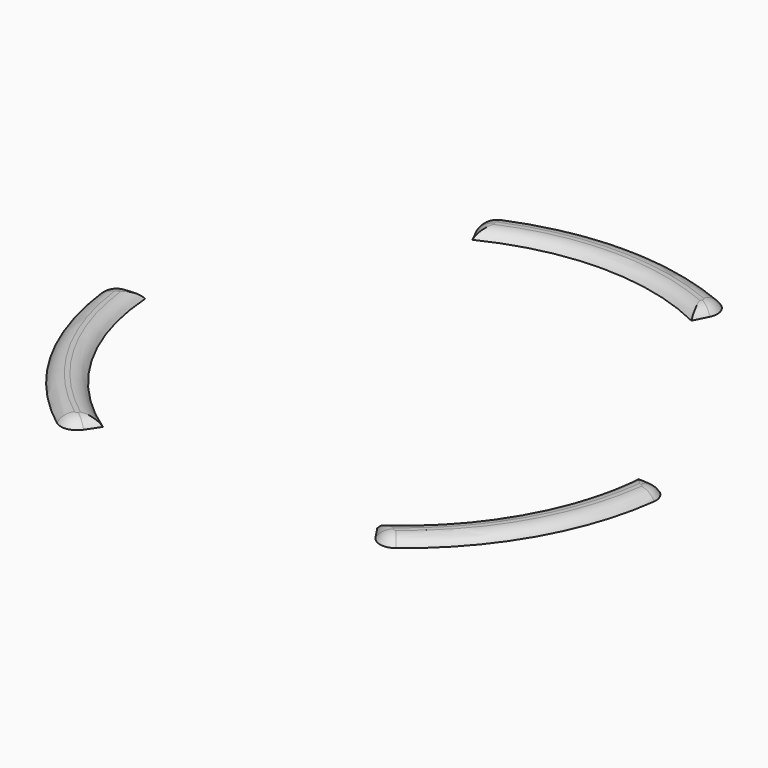
from build123d import *

# Parameters (mm, degrees)
F0_R            = 43.434
F0_R_2          = 38.354
F1_DEPTH        = 1.27
F3_DEPTH        = 25.4
F4_F1_R         = 2.54
F4_F2_R         = 2.54
F4_S1_F1_R      = 2.54
F4_S1_F2_R      = 2.54
F4_S2_F1_R      = 2.54
F4_S2_F2_R      = 2.54
F5_T1_DEPTH     = 7.9603031001
F5_T3_DEPTH     = 7.9603031001
F5_T6_ANGLE     = 45.477927501
F5_T8_ANGLE     = 69.0325853679
F5_T10_ANGLE    = 93.5610362495
F5_T12_ANGLE    = 93.5610362495
F5_S1_T1_DEPTH  = 7.9603031001
F5_S1_T3_DEPTH  = 7.9603031001
F5_S1_T6_ANGLE  = 45.477927501
F5_S1_T8_ANGLE  = 69.0325853679
F5_S1_T10_ANGLE = 93.5610362495
F5_S1_T12_ANGLE = 93.5610362495
F5_S2_T1_DEPTH  = 7.9603031001
F5_S2_T3_DEPTH  = 7.9603031001
F5_S2_T6_ANGLE  = 45.477927501
F5_S2_T8_ANGLE  = 69.0325853679
F5_S2_T10_ANGLE = 93.5610362495
F5_S2_T12_ANGLE = 93.5610362495


# Not quite as in the source:
# - a fillet or chamfer that OpenCascade refuses, or shapes differently, is made with other operations: its cross-section is extruded or revolved along the edge and cut away or added


with BuildPart() as f1:
    # F0 (on Top) → F1 (new body)
    with BuildSketch(Plane.XY):
        Circle(F0_R)
        Circle(F0_R_2, mode=Mode.SUBTRACT)
    extrude(amount=F1_DEPTH)

    # F2 (on Top) → F3 (cut)
    with BuildSketch(Plane.XY):
        Polygon((34.5006046501, -51.7314743282), (0, 0), (-34.5006046501, -51.7314743282), (0, -51.7314743282), align=None)
        Polygon((27.5504686184, 55.744137237), (0, 0), (62.0510732685, -4.0126629088), (44.8007709434, 25.8657371641), align=None)
        Polygon((-62.0510732685, -4.0126629088), (0, 0), (-27.5504686184, 55.744137237), (-44.8007709434, 25.8657371641), align=None)
    extrude(amount=F3_DEPTH, mode=Mode.SUBTRACT)

    # F4: fillet of radius 2.54 on 2 edges, made by hand

    # F4_f1
    f4_f1_edges = [f1.edges().sort_by_distance(p)[0] for p in [
        (-19.2443541023, 38.9379916173, 0.635),
    ]]
    fillet(f4_f1_edges, radius=F4_F1_R)

    # F4_f2
    f4_f2_edges = [f1.edges().sort_by_distance(p)[0] for p in [
        (19.2443541023, 38.9379916173, 0.635),
    ]]
    fillet(f4_f2_edges, radius=F4_F2_R)

    # F4#s1: fillet of radius 2.54 on 2 edges, made by hand

    # F4_s1_f1
    f4_s1_f1_edges = [f1.edges().sort_by_distance(p)[0] for p in [
        (43.343466964, -2.8028962767, 0.635),
    ]]
    fillet(f4_s1_f1_edges, radius=F4_S1_F1_R)

    # F4_s1_f2
    f4_s1_f2_edges = [f1.edges().sort_by_distance(p)[0] for p in [
        (24.0991128618, -36.1350953406, 0.635),
    ]]
    fillet(f4_s1_f2_edges, radius=F4_S1_F2_R)

    # F4#s2: fillet of radius 2.54 on 2 edges, made by hand

    # F4_s2_f1
    f4_s2_f1_edges = [f1.edges().sort_by_distance(p)[0] for p in [
        (-24.0991128618, -36.1350953406, 0.635),
    ]]
    fillet(f4_s2_f1_edges, radius=F4_S2_F1_R)

    # F4_s2_f2
    f4_s2_f2_edges = [f1.edges().sort_by_distance(p)[0] for p in [
        (-43.343466964, -2.8028962767, 0.635),
    ]]
    fillet(f4_s2_f2_edges, radius=F4_S2_F2_R)

    # F5: fillet of radius 2.54 on 2 edges, made by hand

    # F5_s2 → F5_t1 (cut)
    with BuildSketch(Plane(origin=(-22.6459984911, -33.9562422589, 0), x_dir=(0, 0, 1), z_dir=(0.5548444274, 0.8319541221, 0))):
        with BuildLine():
            ThreePointArc((1.27, -2.1997045256), (0.9297045256, -0.9297045256), (0, 0))
            Line((0, 0), (1.27, 0))
            Line((1.27, 0), (1.27, -2.1997045256))
        make_face()
    extrude(amount=F5_T1_DEPTH, mode=Mode.SUBTRACT)

    # F5_s4 → F5_t3 (cut)
    with BuildSketch(Plane(origin=(-32.786256869, -2.1201921245, 0), x_dir=(0, 0, 1), z_dir=(-0.9979156183, -0.0645323083, 0))):
        with BuildLine():
            ThreePointArc((1.27, -2.1997045256), (0.9297045256, -0.9297045256), (0, 0))
            Line((0, 0), (1.27, 0))
            Line((1.27, 0), (1.27, -2.1997045256))
        make_face()
    extrude(amount=F5_T3_DEPTH, mode=Mode.SUBTRACT)

    # F5_s5 → F5_t6 (revolve, cut)
    with BuildSketch(Plane(origin=(0, 0, 0), x_dir=(0, 0, 1), z_dir=(-0.1263900457, 0.991980623, 0))):
        with BuildLine():
            ThreePointArc((0, -43.434), (0.9297045256, -42.5042954744), (1.27, -41.2342954744))
            Line((1.27, -41.2342954744), (1.27, -43.434))
            Line((1.27, -43.434), (0, -43.434))
        make_face()
    revolve(axis=Axis((0, 0, 1.27), (0, 0, 1)), revolution_arc=F5_T6_ANGLE, mode=Mode.SUBTRACT)

    # F5_s7 → F5_t8 (revolve, cut)
    with BuildSketch(Plane(origin=(0, 0, 0), x_dir=(0, 0, 1), z_dir=(0.0787425769, 0.9968949827, 0))):
        with BuildLine():
            ThreePointArc((1.27, -40.5537045256), (0.9297045256, -39.2837045256), (0, -38.354))
            Line((0, -38.354), (1.27, -38.354))
            Line((1.27, -38.354), (1.27, -40.5537045256))
        make_face()
    revolve(axis=Axis((0, 0, 1.27), (0, 0, 1)), revolution_arc=F5_T8_ANGLE, mode=Mode.SUBTRACT)

    # F5_s9 → F5_t10 (revolve, cut)
    with BuildSketch(Plane(origin=(0, 0, 0), x_dir=(0, 0, 1), z_dir=(0.1263900457, -0.991980623, 0))):
        with BuildLine():
            ThreePointArc((0, 43.434), (0.9297045256, 42.5042954744), (1.27, 41.2342954744))
            Line((1.27, 41.2342954744), (1.27, 43.434))
            Line((1.27, 43.434), (0, 43.434))
        make_face()
    revolve(axis=Axis((-40.5660555958, -5.1685945283, 1.27), (0, 0, -1)), revolution_arc=F5_T10_ANGLE, mode=Mode.SUBTRACT)

    # F5_s11 → F5_t12 (revolve, cut)
    with BuildSketch(Plane(origin=(0, 0, 0), x_dir=(0, 0, 1), z_dir=(-0.7958853967, 0.6054473018, 0))):
        with BuildLine():
            ThreePointArc((0, -43.434), (0.9297045256, -42.5042954744), (1.27, -41.2342954744))
            Line((1.27, -41.2342954744), (1.27, -43.434))
            Line((1.27, -43.434), (0, -43.434))
        make_face()
    revolve(axis=Axis((-24.7591619613, -32.5469374131, 1.27), (0, 0, 1)), revolution_arc=F5_T12_ANGLE, mode=Mode.SUBTRACT)

    # F5#s1: fillet of radius 2.54 on 2 edges, made by hand

    # F5_s1_s2 → F5_s1_t1 (cut)
    with BuildSketch(Plane(origin=(40.7299676588, -2.6338888579, 0), x_dir=(0, 0, 1), z_dir=(-0.9979156183, 0.0645323083, 0))):
        with BuildLine():
            ThreePointArc((0, 0), (0.9297045256, -0.9297045256), (1.27, -2.1997045256))
            Line((1.27, -2.1997045256), (1.27, 0))
            Line((1.27, 0), (0, 0))
        make_face()
    extrude(amount=F5_S1_T1_DEPTH, mode=Mode.SUBTRACT)

    # F5_s1_s4 → F5_s1_t3 (cut)
    with BuildSketch(Plane(origin=(18.2292686752, -27.3336352813, 0), x_dir=(0, 0, 1), z_dir=(0.5548444274, -0.8319541221, 0))):
        with BuildLine():
            ThreePointArc((0, 0), (0.9297045256, -0.9297045256), (1.27, -2.1997045256))
            Line((1.27, -2.1997045256), (1.27, 0))
            Line((1.27, 0), (0, 0))
        make_face()
    extrude(amount=F5_S1_T3_DEPTH, mode=Mode.SUBTRACT)

    # F5_s1_s5 → F5_s1_t6 (revolve, cut)
    with BuildSketch(Plane(origin=(0, 0, 0), x_dir=(0, 0, 1), z_dir=(-0.7958853967, -0.6054473018, 0))):
        with BuildLine():
            ThreePointArc((0, -43.434), (0.9297045256, -42.5042954744), (1.27, -41.2342954744))
            Line((1.27, -41.2342954744), (1.27, -43.434))
            Line((1.27, -43.434), (0, -43.434))
        make_face()
    revolve(axis=Axis((0, 0, 1.27), (0, 0, 1)), revolution_arc=F5_S1_T6_ANGLE, mode=Mode.SUBTRACT)

    # F5_s1_s7 → F5_s1_t8 (revolve, cut)
    with BuildSketch(Plane(origin=(0, 0, 0), x_dir=(0, 0, 1), z_dir=(-0.9027076684, -0.4302544194, 0))):
        with BuildLine():
            ThreePointArc((0, -38.354), (0.9297045256, -39.2837045256), (1.27, -40.5537045256))
            Line((1.27, -40.5537045256), (1.27, -38.354))
            Line((1.27, -38.354), (0, -38.354))
        make_face()
    revolve(axis=Axis((0, 0, 1.27), (0, 0, 1)), revolution_arc=F5_S1_T8_ANGLE, mode=Mode.SUBTRACT)

    # F5_s1_s9 → F5_s1_t10 (revolve, cut)
    with BuildSketch(Plane(origin=(0, 0, 0), x_dir=(0, 0, 1), z_dir=(0.7958853967, 0.6054473018, 0))):
        with BuildLine():
            ThreePointArc((0, 43.434), (0.9297045256, 42.5042954744), (1.27, 41.2342954744))
            Line((1.27, 41.2342954744), (1.27, 43.434))
            Line((1.27, 43.434), (0, 43.434))
        make_face()
    revolve(axis=Axis((24.7591619613, -32.5469374131, 1.27), (0, 0, -1)), revolution_arc=F5_S1_T10_ANGLE, mode=Mode.SUBTRACT)

    # F5_s1_s11 → F5_s1_t12 (revolve, cut)
    with BuildSketch(Plane(origin=(0, 0, 0), x_dir=(0, 0, 1), z_dir=(-0.1263900457, -0.991980623, 0))):
        with BuildLine():
            ThreePointArc((0, -43.434), (0.9297045256, -42.5042954744), (1.27, -41.2342954744))
            Line((1.27, -41.2342954744), (1.27, -43.434))
            Line((1.27, -43.434), (0, -43.434))
        make_face()
    revolve(axis=Axis((40.5660555958, -5.1685945283, 1.27), (0, 0, 1)), revolution_arc=F5_S1_T12_ANGLE, mode=Mode.SUBTRACT)

    # F5#s2: fillet of radius 2.54 on 2 edges, made by hand

    # F5_s2_s2 → F5_s2_t1 (cut)
    with BuildSketch(Plane(origin=(-18.0839691677, 36.5901311168, 0), x_dir=(0, 0, 1), z_dir=(0.4430711908, -0.8964864304, 0))):
        with BuildLine():
            ThreePointArc((1.27, -2.1997045256), (0.9297045256, -0.9297045256), (0, 0))
            Line((0, 0), (1.27, 0))
            Line((1.27, 0), (1.27, -2.1997045256))
        make_face()
    extrude(amount=F5_S2_T1_DEPTH, mode=Mode.SUBTRACT)

    # F5_s2_s4 → F5_s2_t3 (cut)
    with BuildSketch(Plane(origin=(14.5569881938, 29.4538274058, 0), x_dir=(0, 0, 1), z_dir=(0.4430711908, 0.8964864304, 0))):
        with BuildLine():
            ThreePointArc((1.27, -2.1997045256), (0.9297045256, -0.9297045256), (0, 0))
            Line((0, 0), (1.27, 0))
            Line((1.27, 0), (1.27, -2.1997045256))
        make_face()
    extrude(amount=F5_S2_T3_DEPTH, mode=Mode.SUBTRACT)

    # F5_s2_s5 → F5_s2_t6 (revolve, cut)
    with BuildSketch(Plane(origin=(0, 0, 0), x_dir=(0, 0, 1), z_dir=(0.9222754424, -0.3865333211, 0))):
        with BuildLine():
            ThreePointArc((0, -43.434), (0.9297045256, -42.5042954744), (1.27, -41.2342954744))
            Line((1.27, -41.2342954744), (1.27, -43.434))
            Line((1.27, -43.434), (0, -43.434))
        make_face()
    revolve(axis=Axis((0, 0, 1.27), (0, 0, 1)), revolution_arc=F5_S2_T6_ANGLE, mode=Mode.SUBTRACT)

    # F5_s2_s7 → F5_s2_t8 (revolve, cut)
    with BuildSketch(Plane(origin=(0, 0, 0), x_dir=(0, 0, 1), z_dir=(0.8239650915, -0.5666405634, 0))):
        with BuildLine():
            ThreePointArc((1.27, -40.5537045256), (0.9297045256, -39.2837045256), (0, -38.354))
            Line((0, -38.354), (1.27, -38.354))
            Line((1.27, -38.354), (1.27, -40.5537045256))
        make_face()
    revolve(axis=Axis((0, 0, 1.27), (0, 0, 1)), revolution_arc=F5_S2_T8_ANGLE, mode=Mode.SUBTRACT)

    # F5_s2_s9 → F5_s2_t10 (revolve, cut)
    with BuildSketch(Plane(origin=(0, 0, 0), x_dir=(0, 0, 1), z_dir=(-0.9222754424, 0.3865333211, 0))):
        with BuildLine():
            ThreePointArc((0, 43.434), (0.9297045256, 42.5042954744), (1.27, 41.2342954744))
            Line((1.27, 41.2342954744), (1.27, 43.434))
            Line((1.27, 43.434), (0, 43.434))
        make_face()
    revolve(axis=Axis((15.8068936345, 37.7155319415, 1.27), (0, 0, -1)), revolution_arc=F5_S2_T10_ANGLE, mode=Mode.SUBTRACT)

    # F5_s2_s11 → F5_s2_t12 (revolve, cut)
    with BuildSketch(Plane(origin=(0, 0, 0), x_dir=(0, 0, 1), z_dir=(0.9222754424, 0.3865333211, 0))):
        with BuildLine():
            ThreePointArc((0, -43.434), (0.9297045256, -42.5042954744), (1.27, -41.2342954744))
            Line((1.27, -41.2342954744), (1.27, -43.434))
            Line((1.27, -43.434), (0, -43.434))
        make_face()
    revolve(axis=Axis((-15.8068936345, 37.7155319415, 1.27), (0, 0, 1)), revolution_arc=F5_S2_T12_ANGLE, mode=Mode.SUBTRACT)


solid = f1.part
